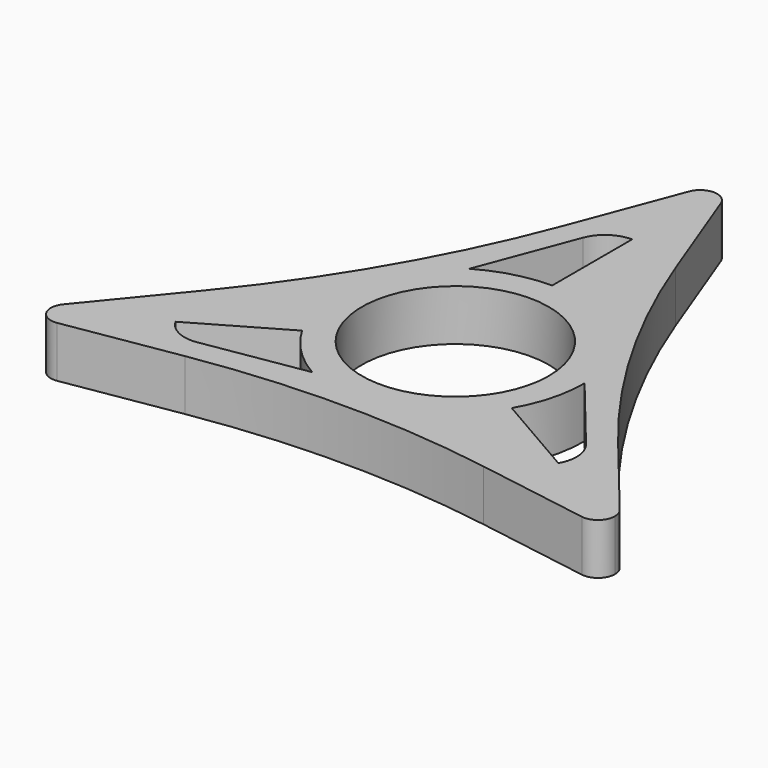
from build123d import *

# Parameters (mm, degrees)
F0_R     = 11
F1_DEPTH = 6


# Not quite as in the source:
# - a feature names something its author has since deleted; it is built from what else it names


with BuildPart() as f1:
    # F0 (on Top) → F1 (new body)
    with BuildSketch(Plane.XY):
        with BuildLine():
            ThreePointArc((1.8708277189, 36.7071093595), (1.9674419226, 36.3594054551), (2, 36))
            ThreePointArc((2, 36), (-0.3594054551, 34.0325580774), (-1.8708277189, 36.7071093595))
            Line((-1.8708277189, 36.7071093595), (-6.6345304801, 24.1035890545))
            ThreePointArc((-6.6345304801, 24.1035890545), (-14.1770019873, 8.1850959137), (-24.1915856836, -6.3061225893))
            Line((-24.1915856836, -6.3061225893), (-32.7247030643, -16.7333703491))
            ThreePointArc((-32.7247030643, -16.7333703491), (-30.5044478293, -16.116442587), (-29.1769145362, -18))
            ThreePointArc((-29.1769145362, -18), (-29.6527625783, -19.2949752156), (-30.8538753454, -19.9737390104))
            Line((-30.8538753454, -19.9737390104), (-17.5570552035, -17.7974664652))
            ThreePointArc((-17.5570552035, -17.7974664652), (0, -16.3701918273), (17.5570552035, -17.7974664652))
            Line((17.5570552035, -17.7974664652), (30.8538753454, -19.9737390104))
            ThreePointArc((30.8538753454, -19.9737390104), (29.4448637287, -17), (32.7247030643, -16.7333703491))
            Line((32.7247030643, -16.7333703491), (24.1915856836, -6.3061225893))
            ThreePointArc((24.1915856836, -6.3061225893), (14.1770019873, 8.1850959137), (6.6345304801, 24.1035890545))
            Line((6.6345304801, 24.1035890545), (1.8708277189, 36.7071093595))
        make_face()
        with BuildLine():
            ThreePointArc((-18.4064805015, -14.9474780208), (-20.765299785, -14.6147639762), (-22.5166604984, -13))
            Line((-22.5166604984, -13), (-12.3317924474, -7.1197636891))
            ThreePointArc((-12.3317924474, -7.1197636891), (-9.7788523145, -10.4437050957), (-6.4502961482, -12.9906255195))
            Line((-6.4502961482, -12.9906255195), (-18.4064805015, -14.9474780208))
        make_face(mode=Mode.SUBTRACT)
        with BuildLine():
            ThreePointArc((22.1481359393, -8.4667406982), (23.0394067662, -10.6758951429), (22.5166604984, -13))
            Line((22.5166604984, -13), (12.3317924474, -7.1197636891))
            ThreePointArc((12.3317924474, -7.1197636891), (13.9339400798, -3.2468819763), (14.4753597851, 0.9091924335))
            Line((14.4753597851, 0.9091924335), (22.1481359393, -8.4667406982))
        make_face(mode=Mode.SUBTRACT)
        Circle(F0_R, mode=Mode.SUBTRACT)
        with BuildLine():
            ThreePointArc((-3.7416554378, 23.414218719), (-2.2741069812, 25.2906591191), (0, 26))
            Line((0, 26), (0, 14.2395273782))
            ThreePointArc((0, 14.2395273782), (-4.1550877653, 13.6905870721), (-8.0250636368, 12.0814330861))
            Line((-8.0250636368, 12.0814330861), (-3.7416554378, 23.414218719))
        make_face(mode=Mode.SUBTRACT)
        with BuildLine():
            ThreePointArc((-1.8708277189, 36.7071093595), (-0.3594054551, 34.0325580774), (2, 36))
            ThreePointArc((2, 36), (1.9674419226, 36.3594054551), (1.8708277189, 36.7071093595))
            ThreePointArc((1.8708277189, 36.7071093595), (0, 38), (-1.8708277189, 36.7071093595))
        make_face()
        with BuildLine():
            ThreePointArc((33.1769145362, -18), (33.0604719492, -17.327533293), (32.7247030643, -16.7333703491))
            ThreePointArc((32.7247030643, -16.7333703491), (29.4448637287, -17), (30.8538753454, -19.9737390104))
            ThreePointArc((30.8538753454, -19.9737390104), (32.4718897519, -19.5241519579), (33.1769145362, -18))
        make_face()
        with BuildLine():
            ThreePointArc((-29.1769145362, -18), (-30.5044478293, -16.116442587), (-32.7247030643, -16.7333703491))
            ThreePointArc((-32.7247030643, -16.7333703491), (-32.9089653438, -19), (-30.8538753454, -19.9737390104))
            ThreePointArc((-30.8538753454, -19.9737390104), (-29.6527625783, -19.2949752156), (-29.1769145362, -18))
        make_face()
    extrude(amount=F1_DEPTH)


solid = f1.part
